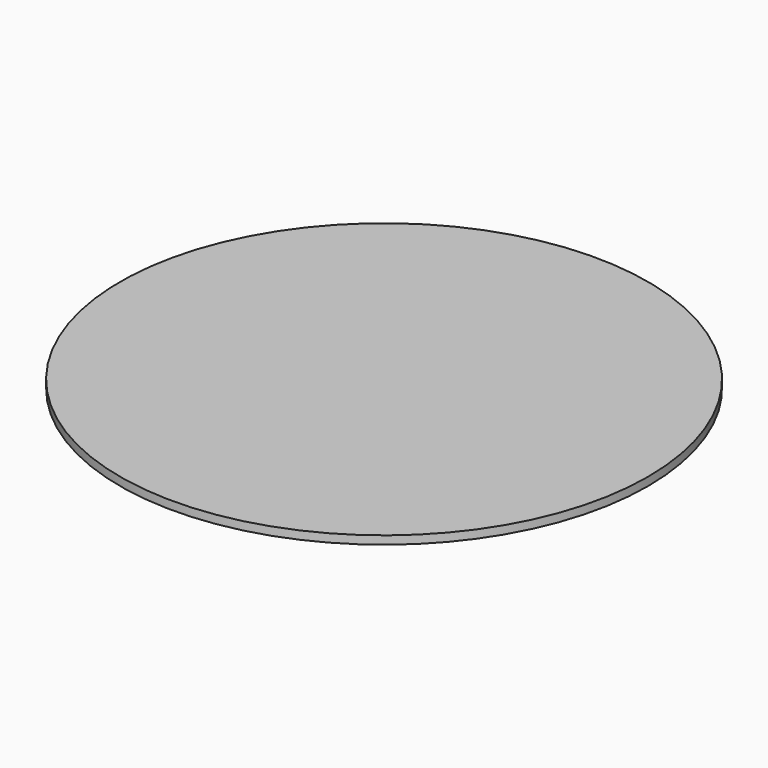
from build123d import *

# Parameters (mm, degrees)
F0_R     = 101.6
F1_DEPTH = 3.175


# Not quite as in the source:
# - a length typed as a fraction of an inch, garbled in the dataset ("3 / 203.2 mm" for 3/8 in), is restored


with BuildPart() as f1:
    # F0 (on Top) → F1 (new body)
    with BuildSketch(Plane.XY):
        Circle(F0_R)
    extrude(amount=F1_DEPTH)


solid = f1.part
